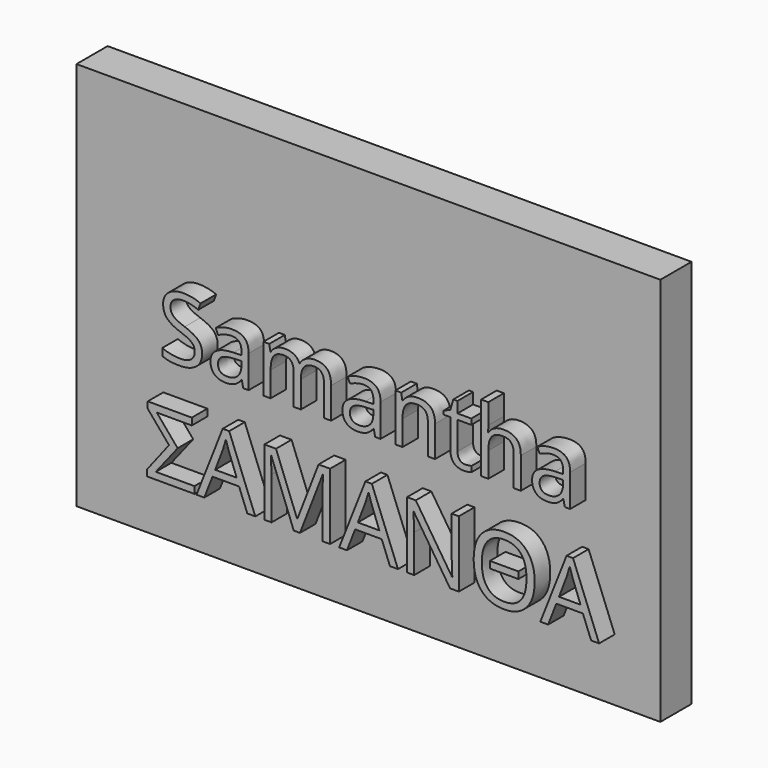
from build123d import *

# Parameters (mm, degrees)
F0_W         = 381
F0_H         = 254
F1_DEPTH     = 25.4
F2_TEXT_SIZE = 57.9196442333
F5_DEPTH     = 12.7
F3_TEXT_SIZE = 60.6186894907
F4_DEPTH     = 12.7


# Not quite as in the source:
# - Text() gives the source's letters only with a copy of the font that has no kerning and outlines rounded to 1/6400 em; it was checked with that copy


with BuildPart() as f1:
    # F0 (on Front) → F1 (new body)
    with BuildSketch(Plane.XZ):
        Rectangle(F0_W, F0_H)
    extrude(amount=F1_DEPTH)

    # F2 (on face) → F5 (join)
    with BuildSketch(Plane.XZ.offset(25.4)):
        with Locations((-127.3551434278, -15.3739005327)):
            Text('Samantha', F2_TEXT_SIZE, font='Open Sans', text_align=(TextAlign.LEFT, TextAlign.BOTTOM))
    extrude(amount=F5_DEPTH)

    # F3 (on face) → F4 (join)
    with BuildSketch(Plane.XZ.offset(25.4)):
        with Locations((-136.389374733, -86.4381939173)):
            Text('ΣΑΜΑΝΘΑ', F3_TEXT_SIZE, font='Open Sans', text_align=(TextAlign.LEFT, TextAlign.BOTTOM))
    extrude(amount=F4_DEPTH)


solid = f1.part
